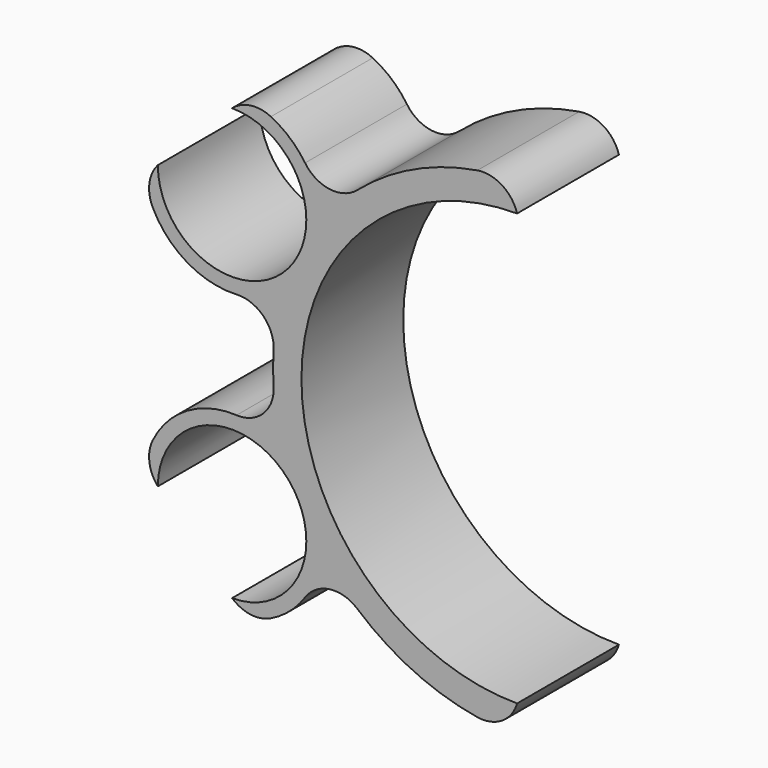
from build123d import *

# Parameters (mm, degrees)
F1_DEPTH     = 18
F2_T1_DEPTH  = 18
F2_T3_DEPTH  = 18
F2_T5_DEPTH  = 18
F2_T7_DEPTH  = 18
F2_T9_DEPTH  = 46.171808491
F2_T11_DEPTH = 46.171808491
F2_T13_DEPTH = 46.171808491
F2_T15_DEPTH = 46.171808491
F2_T17_DEPTH = 46.1730452367
F2_T19_DEPTH = 46.1730452367


# Not quite as in the source:
# - a fillet or chamfer that OpenCascade refuses, or shapes differently, is made with other operations: its cross-section is extruded or revolved along the edge and cut away or added


with BuildPart() as f1:
    # F0 (on Front) → F1 (new body)
    with BuildSketch(Plane.XZ):
        with BuildLine():
            ThreePointArc((-30.9053214059, 15.3333332579), (-29.4709612635, 17.9363441706), (-27.8178919283, 20.4062463149))
            ThreePointArc((-27.8178919283, 20.4062463149), (-31.6172700774, 28.9813161323), (-40.3112887415, 32.5))
            Line((-40.3112887415, 32.5), (-40.3112887415, 30.5))
            ThreePointArc((-40.3112887415, 30.5), (-32.886667539, 27.4246212025), (-29.8112887415, 20))
            ThreePointArc((-29.8112887415, 20), (-30.0884550584, 17.6034041876), (-30.9053214059, 15.3333332579))
        make_face()
        with BuildLine():
            ThreePointArc((0, -30.5), (-30.5, 0), (0, 30.5))
            Line((0, 30.5), (0, 34.5))
            ThreePointArc((0, 34.5), (-15.5922176443, 30.7755219116), (-27.8178919283, 20.4062463149))
            ThreePointArc((-27.8178919283, 20.4062463149), (-27.8129396472, 20.203149988), (-27.8112887415, 20))
            ThreePointArc((-27.8112887415, 20), (-29.205476311, 14.2631951176), (-33.0770375829, 9.8060993641))
            ThreePointArc((-33.0770375829, 9.8060993641), (-34.5, 0), (-33.0770375829, -9.8060993641))
            ThreePointArc((-33.0770375829, -9.8060993641), (-29.205476311, -14.2631951176), (-27.8112887415, -20))
            ThreePointArc((-27.8112887415, -20), (-27.8129396472, -20.203149988), (-27.8178919283, -20.4062463149))
            ThreePointArc((-27.8178919283, -20.4062463149), (-15.5922176443, -30.7755219116), (0, -34.5))
            Line((0, -34.5), (0, -30.5))
        make_face()
        with BuildLine():
            ThreePointArc((-27.8112887415, 20), (-27.8129396472, 20.203149988), (-27.8178919283, 20.4062463149))
            ThreePointArc((-27.8178919283, 20.4062463149), (-29.4709612635, 17.9363441706), (-30.9053214059, 15.3333332579))
            ThreePointArc((-30.9053214059, 15.3333332579), (-32.1103276855, 12.6165310576), (-33.0770375829, 9.8060993641))
            ThreePointArc((-33.0770375829, 9.8060993641), (-29.205476311, 14.2631951176), (-27.8112887415, 20))
        make_face()
        with BuildLine():
            ThreePointArc((-30.905321409, -15.3333332517), (-29.4709612653, -17.9363441676), (-27.8178919283, -20.4062463149))
            ThreePointArc((-27.8178919283, -20.4062463149), (-27.8129396472, -20.203149988), (-27.8112887415, -20))
            ThreePointArc((-27.8112887415, -20), (-29.205476311, -14.2631951176), (-33.0770375829, -9.8060993641))
            ThreePointArc((-33.0770375829, -9.8060993641), (-32.1103276868, -12.6165310544), (-30.905321409, -15.3333332517))
        make_face()
        with BuildLine():
            ThreePointArc((-33.0770375829, 9.8060993641), (-32.1103276855, 12.6165310576), (-30.9053214059, 15.3333332579))
            ThreePointArc((-30.9053214059, 15.3333332579), (-42.7078845539, 9.7771663169), (-50.8112887415, 20))
            Line((-50.8112887415, 20), (-52.8112887415, 20))
            ThreePointArc((-52.8112887415, 20), (-46.0480936239, 8.8941875695), (-33.0770375829, 9.8060993641))
        make_face()
        with BuildLine():
            ThreePointArc((-50.8112887415, -20), (-42.7078845573, -9.7771663177), (-30.905321409, -15.3333332517))
            ThreePointArc((-30.905321409, -15.3333332517), (-32.1103276868, -12.6165310544), (-33.0770375829, -9.8060993641))
            ThreePointArc((-33.0770375829, -9.8060993641), (-46.0480936239, -8.8941875695), (-52.8112887415, -20))
            Line((-52.8112887415, -20), (-50.8112887415, -20))
        make_face()
        with BuildLine():
            ThreePointArc((-40.3112887415, -32.5), (-31.6172700774, -28.9813161323), (-27.8178919283, -20.4062463149))
            ThreePointArc((-27.8178919283, -20.4062463149), (-29.4709612653, -17.9363441676), (-30.905321409, -15.3333332517))
            ThreePointArc((-30.905321409, -15.3333332517), (-30.0884550592, -17.6034041842), (-29.8112887415, -20))
            ThreePointArc((-29.8112887415, -20), (-32.886667539, -27.4246212025), (-40.3112887415, -30.5))
            Line((-40.3112887415, -30.5), (-40.3112887415, -32.5))
        make_face()
    extrude(amount=F1_DEPTH)

    # F2: fillet of radius 5 on 10 edges, made by hand

    # F2_s2 → F2_t1 (join)
    with BuildSketch(Plane.XZ):
        with BuildLine():
            ThreePointArc((-29.9854181156, 27.0446004725), (-26.4995189962, 24.9041460638), (-22.5822762114, 26.0823848816))
            ThreePointArc((-22.5822762114, 26.0823848816), (-25.3593942038, 23.3912617363), (-27.8178919283, 20.4062463149))
            ThreePointArc((-27.8178919283, 20.4062463149), (-28.4286678987, 23.8798610678), (-29.9854181156, 27.0446004725))
        make_face()
    extrude(amount=F2_T1_DEPTH)

    # F2_s4 → F2_t3 (join)
    with BuildSketch(Plane.XZ):
        with BuildLine():
            ThreePointArc((-39.6741951276, 7.5162460883), (-35.861056634, 6.0353637247), (-34.4295655704, 2.2034097738))
            ThreePointArc((-34.4295655704, 2.2034097738), (-33.9666835234, 6.0427154842), (-33.0770375829, 9.8060993641))
            ThreePointArc((-33.0770375829, 9.8060993641), (-36.2124627952, 8.1911208888), (-39.6741951276, 7.5162460883))
        make_face()
    extrude(amount=F2_T3_DEPTH)

    # F2_s6 → F2_t5 (join)
    with BuildSketch(Plane.XZ):
        with BuildLine():
            ThreePointArc((-34.4295655704, -2.2034097738), (-35.861056634, -6.0353637247), (-39.6741951276, -7.5162460883))
            ThreePointArc((-39.6741951276, -7.5162460883), (-36.2124627952, -8.1911208888), (-33.0770375829, -9.8060993641))
            ThreePointArc((-33.0770375829, -9.8060993641), (-33.9666835234, -6.0427154842), (-34.4295655704, -2.2034097738))
        make_face()
    extrude(amount=F2_T5_DEPTH)

    # F2_s8 → F2_t7 (join)
    with BuildSketch(Plane.XZ):
        with BuildLine():
            ThreePointArc((-29.9854181156, -27.0446004725), (-26.4995189962, -24.9041460638), (-22.5822762114, -26.0823848816))
            ThreePointArc((-22.5822762114, -26.0823848816), (-25.3593942038, -23.3912617363), (-27.8178919283, -20.4062463149))
            ThreePointArc((-27.8178919283, -20.4062463149), (-28.4286678987, -23.8798610678), (-29.9854181156, -27.0446004725))
        make_face()
    extrude(amount=F2_T7_DEPTH)

    # F2_s10 → F2_t9 (cut)
    with BuildSketch(Plane.XZ.offset(-14.0859042455)):
        with BuildLine():
            ThreePointArc((-34.8218866889, 31.2301587302), (-37.676903372, 31.6944428559), (-40.3112887415, 30.5))
            Line((-40.3112887415, 30.5), (-40.3112887415, 32.5))
            ThreePointArc((-40.3112887415, 32.5), (-37.4941078924, 32.1784026893), (-34.8218866889, 31.2301587302))
        make_face()
    extrude(amount=F2_T9_DEPTH, mode=Mode.SUBTRACT)

    # F2_s12 → F2_t11 (cut)
    with BuildSketch(Plane.XZ.offset(-14.0859042455)):
        with BuildLine():
            ThreePointArc((-51.5414474717, 14.5105979474), (-52.0057315974, 17.3656146306), (-50.8112887415, 20))
            Line((-50.8112887415, 20), (-52.8112887415, 20))
            ThreePointArc((-52.8112887415, 20), (-52.4896914308, 17.1828191509), (-51.5414474717, 14.5105979474))
        make_face()
    extrude(amount=F2_T11_DEPTH, mode=Mode.SUBTRACT)

    # F2_s14 → F2_t13 (cut)
    with BuildSketch(Plane.XZ.offset(-14.0859042455)):
        with BuildLine():
            ThreePointArc((-50.8112887415, -20), (-52.0057315974, -17.3656146306), (-51.5414474717, -14.5105979474))
            ThreePointArc((-51.5414474717, -14.5105979474), (-52.4896914308, -17.1828191509), (-52.8112887415, -20))
            Line((-52.8112887415, -20), (-50.8112887415, -20))
        make_face()
    extrude(amount=F2_T13_DEPTH, mode=Mode.SUBTRACT)

    # F2_s16 → F2_t15 (cut)
    with BuildSketch(Plane.XZ.offset(-14.0859042455)):
        with BuildLine():
            ThreePointArc((-34.8218866889, -31.2301587302), (-37.676903372, -31.6944428559), (-40.3112887415, -30.5))
            Line((-40.3112887415, -30.5), (-40.3112887415, -32.5))
            ThreePointArc((-40.3112887415, -32.5), (-37.4941078924, -32.1784026893), (-34.8218866889, -31.2301587302))
        make_face()
    extrude(amount=F2_T15_DEPTH, mode=Mode.SUBTRACT)

    # F2_s18 → F2_t17 (cut)
    with BuildSketch(Plane.XZ.offset(-14.0865226184)):
        with BuildLine():
            ThreePointArc((0, -30.5), (-2.1356819659, -33.3363611882), (-5.6157903729, -34.0398721867))
            ThreePointArc((-5.6157903729, -34.0398721867), (-2.8173045237, -34.3847756314), (0, -34.5))
            Line((0, -34.5), (0, -30.5))
        make_face()
    extrude(amount=F2_T17_DEPTH, mode=Mode.SUBTRACT)

    # F2_s20 → F2_t19 (cut)
    with BuildSketch(Plane.XZ.offset(-14.0865226184)):
        with BuildLine():
            ThreePointArc((-5.6157903729, 34.0398721867), (-2.1356819659, 33.3363611882), (0, 30.5))
            Line((0, 30.5), (0, 34.5))
            ThreePointArc((0, 34.5), (-2.8173045237, 34.3847756314), (-5.6157903729, 34.0398721867))
        make_face()
    extrude(amount=F2_T19_DEPTH, mode=Mode.SUBTRACT)


solid = f1.part
